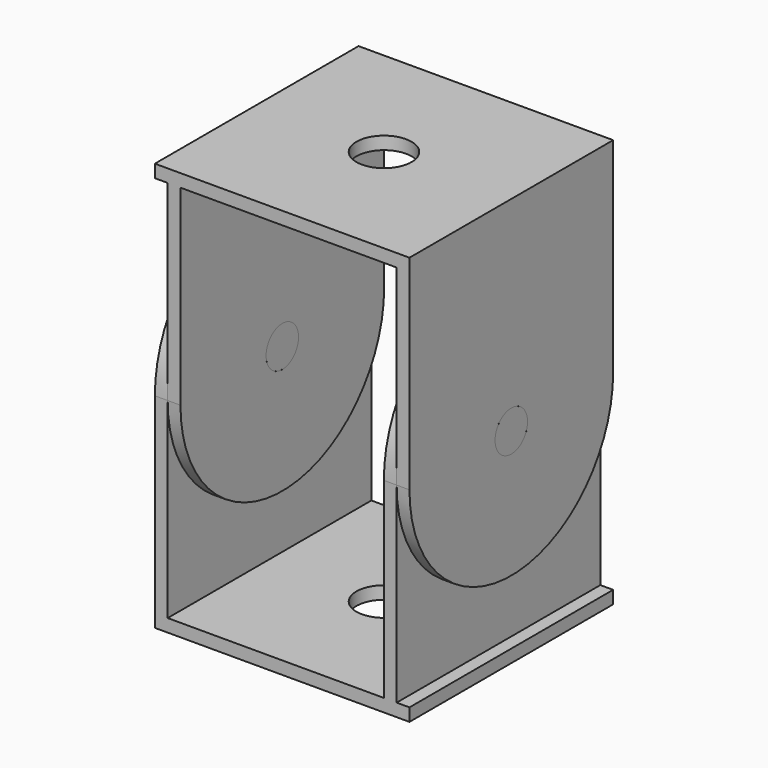
from build123d import *

# Parameters (mm, degrees)
F0_W      = 39.878
F0_H      = 39.878
F0_R      = 4.318
F1_DEPTH  = 2.0066
F5_R      = 3.175
F6_DEPTH  = 2.0066
F7_R      = 3.175
F8_DEPTH  = 2.0066
F9_R      = 3.175
F10_DEPTH = 2.0066
F11_R     = 3.175
F12_DEPTH = 2.0066
F13_R     = 3.175
F14_DEPTH = 4.0132


with BuildPart() as f1:
    # F0 (on Top) → F1 (new body)
    with BuildSketch(Plane.XY):
        Rectangle(F0_W, F0_H)
        Circle(F0_R, mode=Mode.SUBTRACT)
    extrude(amount=F1_DEPTH)


with BuildPart() as f4_1:
    # F4: instance of F1
    add(f1.part.mirror(Plane.XY.offset(32.004)))

    # F5 (on face) → F6 (join)
    with BuildSketch(Plane.YZ.offset(19.939)):
        with BuildLine():
            Line((-19.939, 62.0014), (-19.939, 32.004))
            ThreePointArc((-19.939, 32.004), (0, 12.065), (19.939, 32.004))
            Line((19.939, 32.004), (19.939, 62.0014))
            Line((19.939, 62.0014), (-19.939, 62.0014))
        make_face()
        with Locations((0, 32.004)):
            Circle(F5_R, mode=Mode.SUBTRACT)
    extrude(amount=-F6_DEPTH)

    # F11 (on face) → F12 (join)
    with BuildSketch(Plane.YZ.offset(-17.9324)):
        with BuildLine():
            Line((19.939, 32.004), (19.939, 64.008))
            Line((19.939, 64.008), (-19.939, 64.008))
            Line((-19.939, 64.008), (-19.939, 32.004))
            ThreePointArc((-19.939, 32.004), (0, 12.065), (19.939, 32.004))
        make_face()
        with Locations((0, 32.004)):
            Circle(F11_R, mode=Mode.SUBTRACT)
    extrude(amount=F12_DEPTH)


with BuildPart() as f1_1:
    add(f1.part)

    # F7 (on face) → F8 (join)
    with BuildSketch(Plane(origin=(17.9324, 0, 0), x_dir=(0, -1, 0), z_dir=(-1, 0, 0))):
        with BuildLine():
            Line((-19.939, 32.004), (-19.939, 2.0066))
            Line((-19.939, 2.0066), (19.939, 2.0066))
            Line((19.939, 2.0066), (19.939, 32.004))
            ThreePointArc((19.939, 32.004), (0, 51.943), (-19.939, 32.004))
        make_face()
        with Locations((0, 32.004)):
            Circle(F7_R, mode=Mode.SUBTRACT)
    extrude(amount=F8_DEPTH)

    # F9 (on face) → F10 (join)
    with BuildSketch(Plane(origin=(-19.939, 0, 0), x_dir=(0, -1, 0), z_dir=(-1, 0, 0))):
        with BuildLine():
            Line((-19.939, 2.0066), (19.939, 2.0066))
            Line((19.939, 2.0066), (19.939, 32.004))
            ThreePointArc((19.939, 32.004), (0, 51.943), (-19.939, 32.004))
            Line((-19.939, 32.004), (-19.939, 2.0066))
        make_face()
        with Locations((0, 32.004)):
            Circle(F9_R, mode=Mode.SUBTRACT)
    extrude(amount=-F10_DEPTH)


with BuildPart() as f14:
    # F13 (on face) → F14 (new body, through all)
    with BuildSketch(Plane(origin=(-19.939, 0, 0), x_dir=(0, -1, 0), z_dir=(-1, 0, 0))):
        with Locations((0, 32.004)):
            Circle(F13_R)
    extrude(amount=-F14_DEPTH)


with BuildPart() as f15_1:
    # F15: instance of F14
    add(f14.part.mirror(Plane.YZ))


solid = Compound([f4_1.part, f1_1.part, f14.part, f15_1.part])
